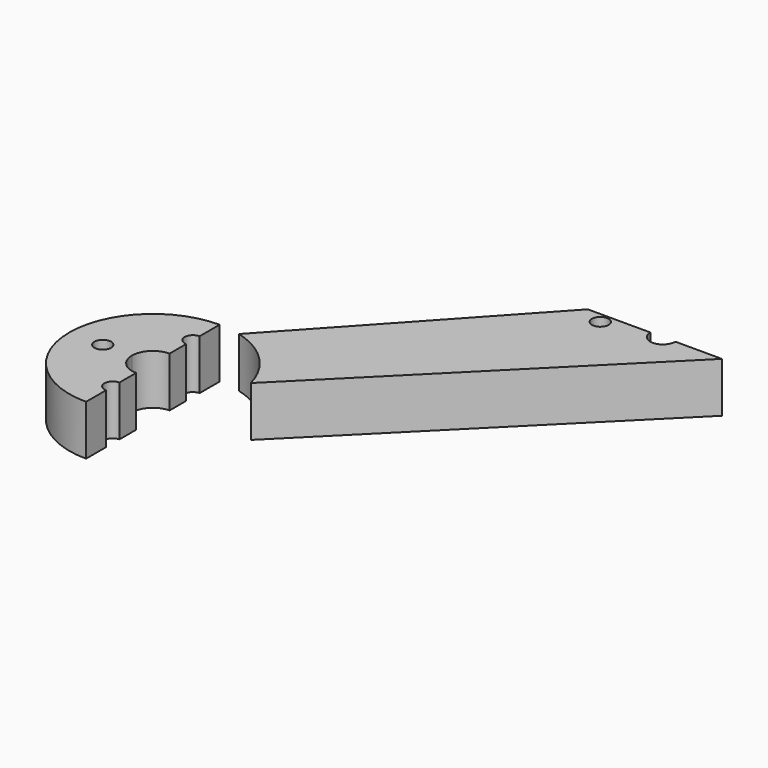
from build123d import *

# Parameters (mm, degrees)
F1_DEPTH = 6


# Not quite as in the source:
# - a feature names something its author has since deleted; it is built from what else it names


with BuildPart() as f1:
    # F0 (on Top) → F1 (new body)
    with BuildSketch(Plane.XY):
        with BuildLine():
            ThreePointArc((-16.3106601718, -16.3106601718), (-16.6358192988, -15.8240251485), (-16.75, -15.25))
            Line((-16.75, -15.25), (-24.25, -15.25))
            Line((-24.25, -15.25), (-46.6029350459, -39.5318672341))
            ThreePointArc((-46.6029350459, -39.5318672341), (-44.191125497, -40.5308714591), (-42.1200576851, -42.1200576851))
            Line((-42.1200576851, -42.1200576851), (-16.3106601718, -16.3106601718))
        make_face()
        with BuildLine():
            ThreePointArc((-22.75, -16.5), (-21.75, -15.5), (-20.75, -16.5))
            ThreePointArc((-20.75, -16.5), (-21.75, -17.5), (-22.75, -16.5))
        make_face(mode=Mode.SUBTRACT)
        with BuildLine():
            Line((-8.1789321881, -15.25), (-13.75, -15.25))
            ThreePointArc((-13.75, -15.25), (-14.6759748515, -16.6358192988), (-16.3106601718, -16.3106601718))
            Line((-16.3106601718, -16.3106601718), (-42.1200576851, -42.1200576851))
            ThreePointArc((-42.1200576851, -42.1200576851), (-40.5308714591, -44.191125497), (-39.5318672341, -46.6029350459))
            Line((-39.5318672341, -46.6029350459), (-8.1789321881, -15.25))
        make_face()
    extrude(amount=F1_DEPTH)


with BuildPart() as f1b:
    # F0 (on Top) → F1, piece 2 (new body)
    with BuildSketch(Plane.XY):
        with BuildLine():
            Line((-49.191125497, -42.191125497), (-49.191125497, -39.191125497))
            ThreePointArc((-49.191125497, -39.191125497), (-56.2621933088, -42.1200576851), (-59.191125497, -49.191125497))
            Line((-59.191125497, -49.191125497), (-56.191125497, -49.191125497))
            ThreePointArc((-56.191125497, -49.191125497), (-55.191125497, -48.191125497), (-54.191125497, -49.191125497))
            Line((-54.191125497, -49.191125497), (-51.691125497, -49.191125497))
            ThreePointArc((-51.691125497, -49.191125497), (-50.9588924499, -47.423358544), (-49.191125497, -46.691125497))
            Line((-49.191125497, -46.691125497), (-49.191125497, -44.191125497))
            ThreePointArc((-49.191125497, -44.191125497), (-50.191125497, -43.191125497), (-49.191125497, -42.191125497))
        make_face()
        with BuildLine():
            Line((-56.191125497, -49.191125497), (-59.191125497, -49.191125497))
            ThreePointArc((-59.191125497, -49.191125497), (-56.2621933088, -56.2621933088), (-49.191125497, -59.191125497))
            Line((-49.191125497, -59.191125497), (-49.191125497, -56.191125497))
            ThreePointArc((-49.191125497, -56.191125497), (-50.191125497, -55.191125497), (-49.191125497, -54.191125497))
            Line((-49.191125497, -54.191125497), (-49.191125497, -51.691125497))
            ThreePointArc((-49.191125497, -51.691125497), (-50.9588924499, -50.9588924499), (-51.691125497, -49.191125497))
            Line((-51.691125497, -49.191125497), (-54.191125497, -49.191125497))
            ThreePointArc((-54.191125497, -49.191125497), (-55.191125497, -50.191125497), (-56.191125497, -49.191125497))
        make_face()
    extrude(amount=F1_DEPTH)


solid = Compound([f1.part, f1b.part])
